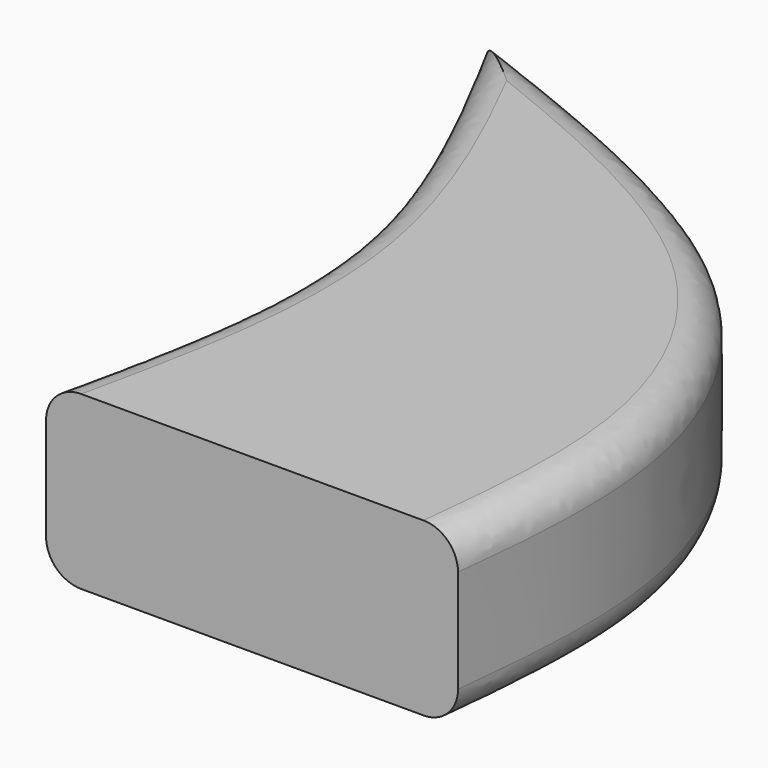
from build123d import *

# Parameters (mm, degrees)
F1_DEPTH = 25
F2_R     = 5


with BuildPart() as f1:
    # F0 (on Top) → F1 (new body)
    with BuildSketch(Plane.XY):
        with BuildLine():
            add(Edge.make_bspline(
                [(-85.2232245209, 89.3407093361), (-76.1078356744, 72.1294474685), (-58.4008853366, 38.8287239467), (-65.7688178685, 5.4617543863), (-69.2891548347, -10.6592906639)],
                knots=[0, 0, 0, 0, 0.5170291798, 1, 1, 1, 1], degree=3))
            Line((-69.2891548347, -10.6592906639), (-9.2891548347, -10.6592906639))
            add(Edge.make_bspline(
                [(-9.2891548347, -10.6592906639), (-7.9778926841, 1.7168816499), (-5.5924427944, 26.9387503571), (-26.6930073641, 67.0668752818), (-64.5008126009, 81.3490670792), (-85.2232245209, 89.3407093361)],
                knots=[0, 0, 0, 0, 0.2984501918, 0.6121588163, 1, 1, 1, 1], degree=3))
        make_face()
    extrude(amount=F1_DEPTH)

    # F2
    f2_edges = [f1.edges().sort_by_distance(p)[0] for p in [
        (-24.084817, 55.731456, 0),
        (-24.084817, 55.731456, 25),
        (-65.088817, 41.176691, 25),
        (-65.088817, 41.176691, 0),
    ]]
    fillet(f2_edges, radius=F2_R)


solid = f1.part
